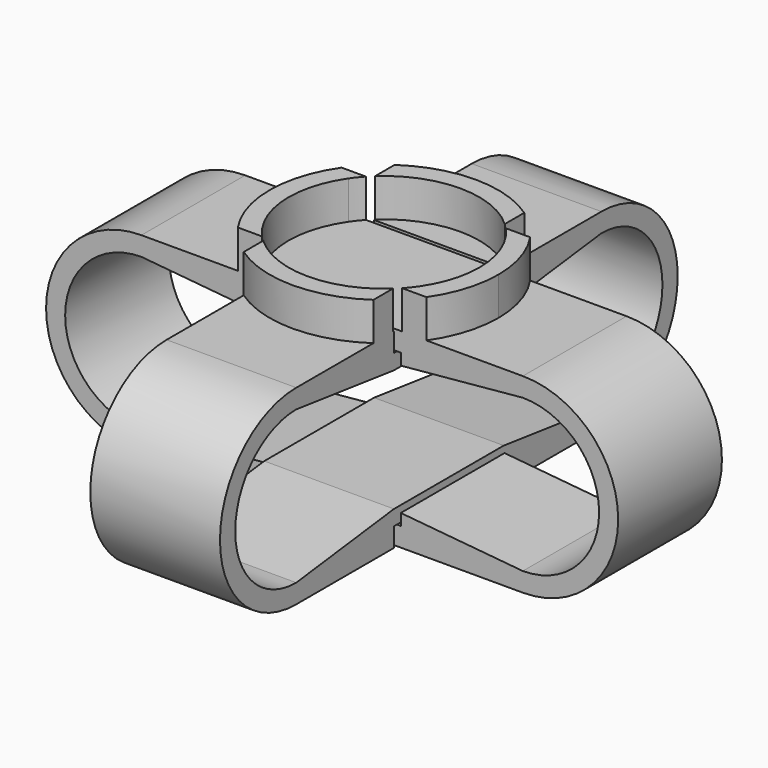
from build123d import *

# Parameters (mm, degrees)
F1_DEPTH      = 8.5
F1_DEPTH_BACK = 8.5
F3_DEPTH      = 8.5
F3_DEPTH_BACK = 8.5
F5_DEPTH      = 5
F6_DEPTH      = 5


# Not quite as in the source:
# - a feature of the source that left no trace in its solid (it failed there, or was rolled back) is left out


with BuildPart() as f1:
    # F0 (on Front) → F1 (new body, two sides)
    with BuildSketch(Plane.XZ) as f1_sk:
        with BuildLine():
            Line((25, 12.5), (-25, 12.5))
            ThreePointArc((-25, 12.5), (-37.5, 0), (-25, -12.5))
            Line((-25, -12.5), (25, -12.5))
            ThreePointArc((25, -12.5), (37.5, 0), (25, 12.5))
        make_face()
        with BuildLine():
            ThreePointArc((-25, -10), (-35, 0), (-25, 10))
            Line((-25, 10), (-9, 8.5))
            Line((-9, 8.5), (-9, 10))
            Line((-9, 10), (9, 10))
            Line((9, 10), (9, 8.5))
            Line((9, 8.5), (25, 10))
            ThreePointArc((25, 10), (35, 0), (25, -10))
            Line((25, -10), (9, -8.5))
            Line((9, -8.5), (9, -10))
            Line((9, -10), (-9, -10))
            Line((-9, -10), (-9, -8.5))
            Line((-9, -8.5), (-25, -10))
        make_face(mode=Mode.SUBTRACT)
    extrude(amount=F1_DEPTH)
    extrude(f1_sk.sketch, amount=-F1_DEPTH_BACK)

    # F4 (on face) → F5 (join)
    with BuildSketch(Plane.XY.offset(12.5)):
        with BuildLine():
            ThreePointArc((-10.2993392453, -7.0833333333), (-12.5, 0), (-10.2993392453, 7.0833333333))
            Line((-10.2993392453, 7.0833333333), (-12.3592070943, 8.5))
            ThreePointArc((-12.3592070943, 8.5), (-15, 0), (-12.3592070943, -8.5))
            Line((-12.3592070943, -8.5), (-10.2993392453, -7.0833333333))
        make_face()
        with BuildLine():
            ThreePointArc((10.2993392453, 7.0833333333), (11.9371634102, 3.7086560527), (12.5, 0))
            ThreePointArc((12.5, 0), (11.9371634102, -3.7086560527), (10.2993392453, -7.0833333333))
            Line((10.2993392453, -7.0833333333), (12.3592070943, -8.5))
            ThreePointArc((12.3592070943, -8.5), (14.3245960923, -4.4503872632), (15, 0))
            ThreePointArc((15, 0), (14.3245960923, 4.4503872632), (12.3592070943, 8.5))
            Line((12.3592070943, 8.5), (10.2993392453, 7.0833333333))
        make_face()
        with BuildLine():
            ThreePointArc((-10.2993392453, 7.0833333333), (-9.7579882677, 7.8122765547), (-9.1651513899, 8.5))
            Line((-9.1651513899, 8.5), (-12.3592070943, 8.5))
            Line((-12.3592070943, 8.5), (-10.2993392453, 7.0833333333))
        make_face()
        with BuildLine():
            ThreePointArc((9.1651513899, 8.5), (9.7579882677, 7.8122765547), (10.2993392453, 7.0833333333))
            Line((10.2993392453, 7.0833333333), (12.3592070943, 8.5))
            Line((12.3592070943, 8.5), (9.1651513899, 8.5))
        make_face()
        with BuildLine():
            Line((12.3592070943, -8.5), (10.2993392453, -7.0833333333))
            ThreePointArc((10.2993392453, -7.0833333333), (9.7579882677, -7.8122765547), (9.1651513899, -8.5))
            Line((9.1651513899, -8.5), (12.3592070943, -8.5))
        make_face()
        with BuildLine():
            ThreePointArc((-9.1651513899, -8.5), (-9.7579882677, -7.8122765547), (-10.2993392453, -7.0833333333))
            Line((-10.2993392453, -7.0833333333), (-12.3592070943, -8.5))
            Line((-12.3592070943, -8.5), (-9.1651513899, -8.5))
        make_face()
    extrude(amount=F5_DEPTH)


with BuildPart() as f3:
    # F2 (on Right) → F3 (new body, two sides)
    with BuildSketch(Plane.YZ) as f3_sk:
        with BuildLine():
            Line((-9, 12.5), (-25, 12.5))
            ThreePointArc((-25, 12.5), (-37.5, 0), (-25, -12.5))
            Line((-25, -12.5), (-9, -12.5))
            Line((-9, -12.5), (-9, -10))
            Line((-9, -10), (9, -10))
            Line((9, -10), (9, -12.5))
            Line((9, -12.5), (25, -12.5))
            ThreePointArc((25, -12.5), (37.5, 0), (25, 12.5))
            Line((25, 12.5), (9, 12.5))
            Line((9, 12.5), (9, 10))
            Line((9, 10), (-9, 10))
            Line((-9, 10), (-9, 12.5))
        make_face()
        with BuildLine():
            ThreePointArc((-25, -10), (-35, 0), (-25, 10))
            Line((-25, 10), (-9, 8))
            Line((-9, 8), (9, 8))
            Line((9, 8), (25, 10))
            ThreePointArc((25, 10), (35, 0), (25, -10))
            Line((25, -10), (9, -8))
            Line((9, -8), (-9, -8))
            Line((-9, -8), (-25, -10))
        make_face(mode=Mode.SUBTRACT)
    extrude(amount=F3_DEPTH)
    extrude(f3_sk.sketch, amount=-F3_DEPTH_BACK)

    # F4 (on face) → F6 (join)
    with BuildSketch(Plane.XY.offset(12.5)):
        with BuildLine():
            ThreePointArc((-8.5, 9.1651513899), (0, 12.5), (8.5, 9.1651513899))
            Line((8.5, 9.1651513899), (8.5, 12.3592070943))
            ThreePointArc((8.5, 12.3592070943), (0, 15), (-8.5, 12.3592070943))
            Line((-8.5, 12.3592070943), (-8.5, 9.1651513899))
        make_face()
        with BuildLine():
            Line((8.5, -12.3592070943), (8.5, -9.1651513899))
            ThreePointArc((8.5, -9.1651513899), (0, -12.5), (-8.5, -9.1651513899))
            Line((-8.5, -9.1651513899), (-8.5, -12.3592070943))
            ThreePointArc((-8.5, -12.3592070943), (0, -15), (8.5, -12.3592070943))
        make_face()
    extrude(amount=F6_DEPTH)


solid = Compound([f1.part, f3.part])
